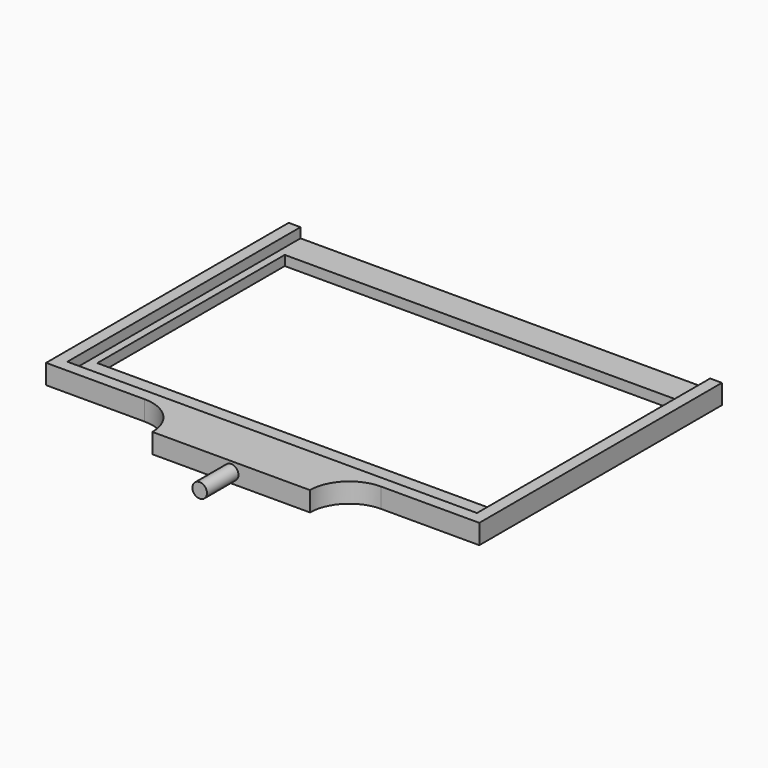
from build123d import *

# Parameters (mm, degrees)
F0_W     = 100.0000001118
F0_H     = 59.5
F0_W_2   = 40
F0_H_2   = 10
F1_DEPTH = 5
F2_W     = 104
F2_H     = 74
F2_W_2   = 100.0000001118
F2_H_2   = 59.5
F3_DEPTH = 2.5
F4_R     = 1.85
F5_DEPTH = 10
F6_R     = 9.99999


# Not quite as in the source:
# - a fillet or chamfer is up to 0.001 mm smaller than in the source, because OpenCascade refuses the exact size


with BuildPart() as f1:
    # F0 (on Top) → F1 (new body)
    with BuildSketch(Plane.XY):
        Polygon((-55, 77), (-55, 0), (-20, 0), (20, 0), (55, 0), (55, 77), align=None)
        with Locations((5.59e-08, 39.75)):
            Rectangle(F0_W, F0_H, mode=Mode.SUBTRACT)
        with Locations((0, -5)):
            Rectangle(F0_W_2, F0_H_2)
    extrude(amount=F1_DEPTH)

    # F2 (on face) → F3 (cut)
    with BuildSketch(Plane.XY.offset(5)):
        with Locations((0, 40)):
            Rectangle(F2_W, F2_H)
        with Locations((5.59e-08, 39.75)):
            Rectangle(F2_W_2, F2_H_2, mode=Mode.SUBTRACT)
    extrude(amount=-F3_DEPTH, mode=Mode.SUBTRACT)

    # F4 (on face) → F5 (join)
    with BuildSketch(Plane.XZ.offset(10)):
        with Locations((0, 2.5)):
            Circle(F4_R)
    extrude(amount=F5_DEPTH)

    # F6 (radius 10 in the source; OpenCascade refuses exactly that, so slightly less here)
    f6_edges = [f1.edges().sort_by_distance(p)[0] for p in [
        (20, 0, 2.5),
        (-20, 0, 2.5),
    ]]
    fillet(f6_edges, radius=F6_R)


solid = f1.part
